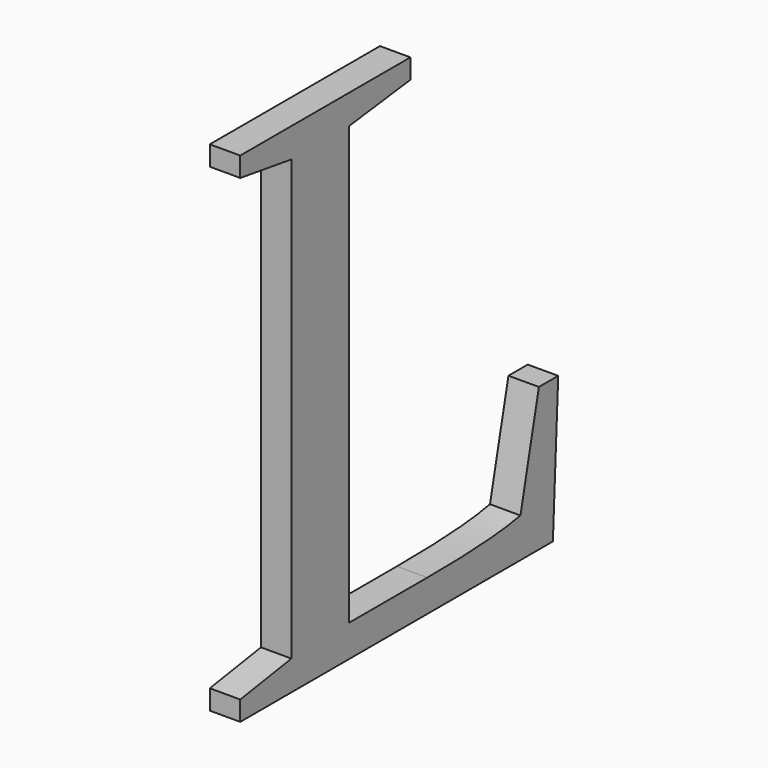
from build123d import *

# Parameters (mm, degrees)
F0_TEXT_SIZE = 635
F1_DEPTH     = 25.4


# Not quite as in the source:
# - Text() gives the source's letters only with a copy of the font that has no kerning and outlines rounded to 1/6400 em; it was checked with that copy


with BuildPart() as f1:
    # F0 (on Right) → F1 (new body)
    with BuildSketch(Plane.YZ):
        with Locations((-349.74609375, 0)):
            Text('L', F0_TEXT_SIZE, font='Tinos', text_align=(TextAlign.LEFT, TextAlign.BOTTOM))
    extrude(amount=F1_DEPTH)


solid = f1.part
